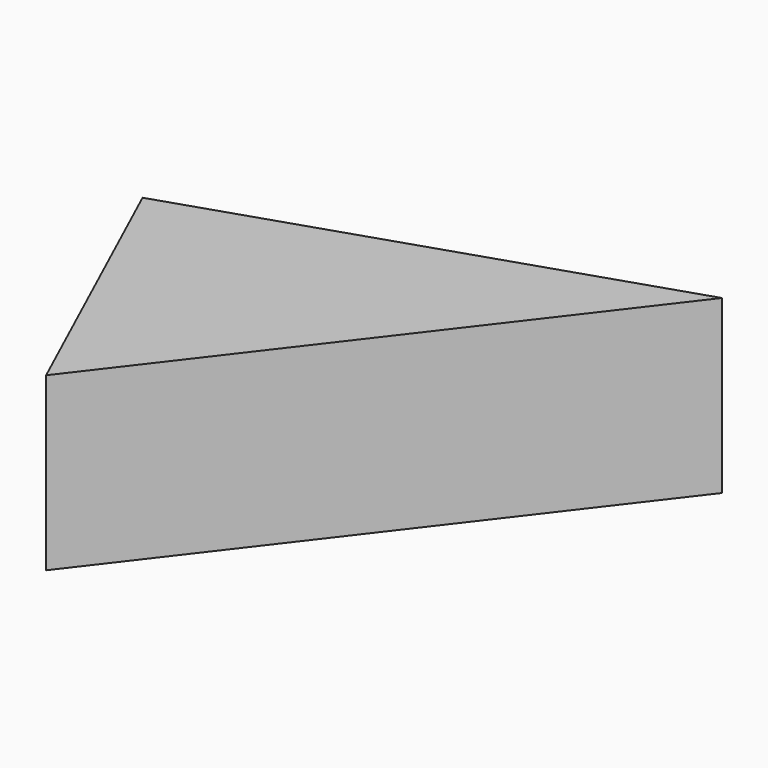
from build123d import *

# Parameters (mm, degrees)
F1_DEPTH = 30


# Not quite as in the source:
# - the program builds the solid bodies; features that only make, move or delete a surface that nothing else refers to are left out


with BuildPart() as f1:
    # F0 (on Top) → F1 (new body)
    with BuildSketch(Plane.XY):
        Polygon((41.2444770336, 39.1447469592), (-38.9947444201, 12.8982812166), (-16.4977610111, -36.2951159477), align=None)
    extrude(amount=F1_DEPTH)


solid = f1.part
